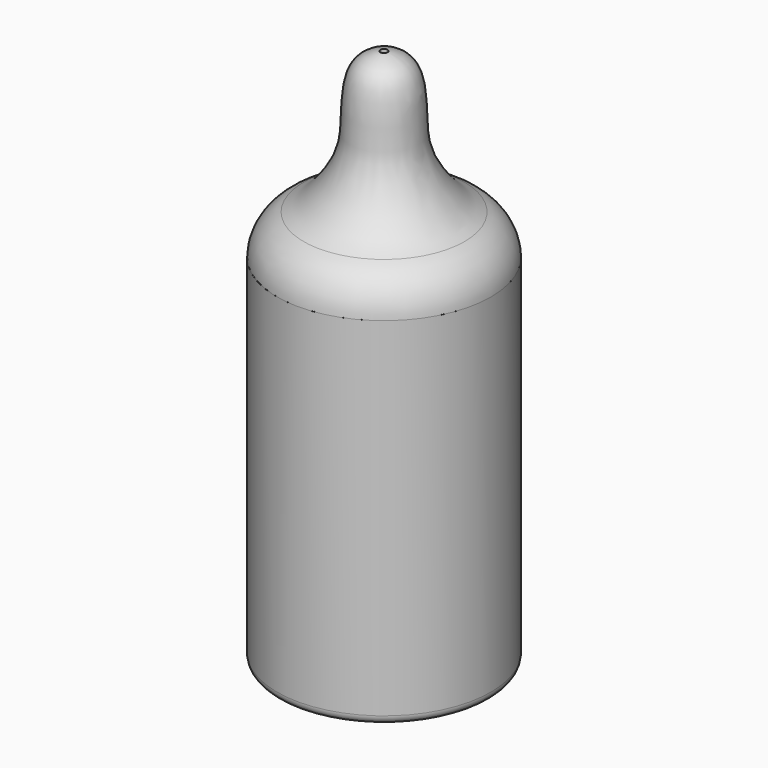
from build123d import *

# Parameters (mm, degrees)
F4_R     = 1.27
F6_R     = 0.508
F7_DEPTH = 2540


with BuildPart() as f1:
    # F0 (on Front) → F1 (revolve)
    with BuildSketch(Plane.XZ):
        with BuildLine():
            Line((0.0129888206, 38.0891347453), (0.0129888206, 14.7824911401))
            Line((0.0129888206, 14.7824911401), (6.35, 14.7824911401))
            ThreePointArc((6.35, 14.7824911401), (10.8401280605, 12.9226192006), (12.7, 8.4324911401))
            Line((12.7, 8.4324911401), (12.7, 0))
            Line((12.7, 0), (13.97, 0))
            Line((13.97, 0), (13.97, 12.1643003333))
            Line((13.97, 12.1643003333), (15.24, 12.1643003333))
            ThreePointArc((15.24, 12.1643003333), (14.1861096276, 15.570023473), (11.4631301434, 17.8711140296))
            add(Edge.make_bspline(
                [(0.0129888206, 38.0891347453), (3.2375221603, 37.7856792591), (5.1139625625, 34.0491835059), (4.5409913214, 26.8386946553), (6.510569033, 22.5911322118), (8.9457915552, 19.5750505607), (10.5066207336, 18.2949238879), (11.4631301434, 17.8711140296)],
                knots=[0, 0, 0, 0, 0.2090800805, 0.4310776593, 0.6112256598, 0.7817355895, 0.8922493546, 0.8922493546, 0.8922493546, 0.8922493546], degree=3))
        make_face()
    revolve(axis=Axis((0.0129888206, 0, 26.4358129427), (0, 0, 1)))

    # F6 (on offset) → F7 (cut)
    with BuildSketch(Plane.XY.offset(38.1)):
        Circle(F6_R)
    extrude(amount=-F7_DEPTH, mode=Mode.SUBTRACT)


with BuildPart() as f3:
    # F2 (on Right) → F3 (revolve)
    with BuildSketch(Plane.YZ):
        Polygon((-15.2270111794, -38.6356996667), (0, -38.6356996667), (0, -36.0956996667), (-14.2110111794, -36.0956996667), (-14.2110111794, 12.1643003333), (-15.2270111794, 12.1643003333), align=None)
    revolve(axis=Axis((0, 0, -37.3656996667), (0, 0, 1)))

    # F4
    f4_edges = [f3.edges().sort_by_distance(p)[0] for p in [
        (0, 15.227011, -38.6357),
    ]]
    fillet(f4_edges, radius=F4_R)


solid = Compound([f1.part, f3.part])
